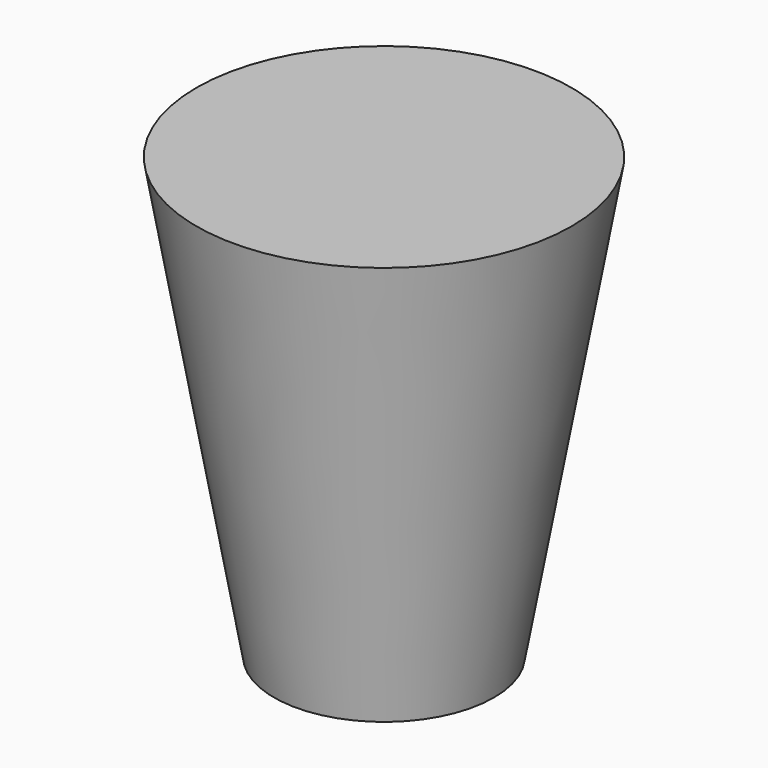
from build123d import *

# Parameters (mm, degrees)
F0_R     = 50
F1_DEPTH = 200
F1_TAPER = -10


with BuildPart() as f1:
    # F0 (on Top) → F1 (new body)
    with BuildSketch(Plane.XY):
        Circle(F0_R)
    extrude(amount=F1_DEPTH, taper=F1_TAPER)


solid = f1.part
